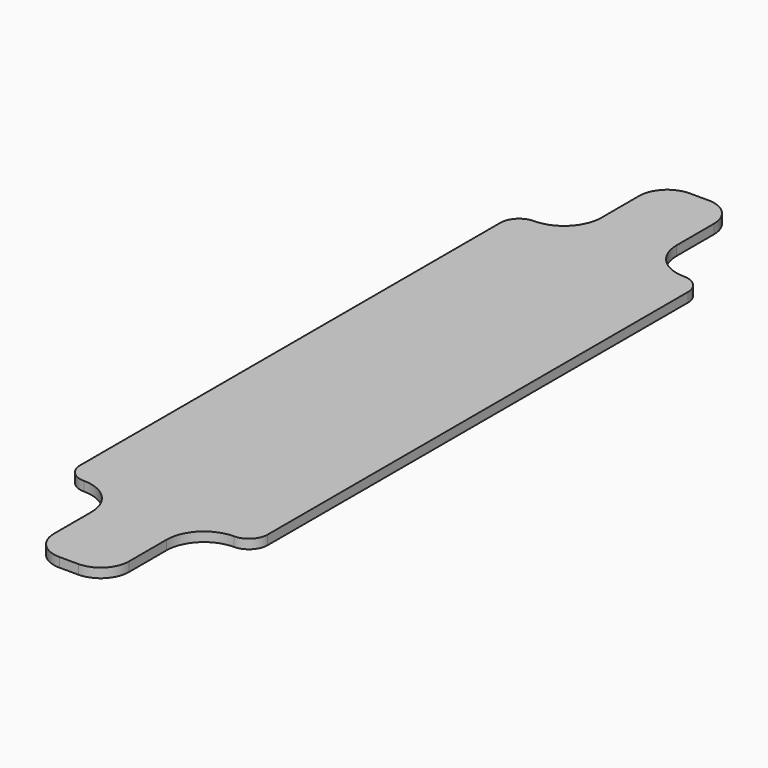
from build123d import *

# Parameters (mm, degrees)
F1_DEPTH = 12.7
F2_R     = 50.8
F3_R     = 38.1
F4_R     = 25.39999


# Not quite as in the source:
# - a fillet or chamfer is up to 0.001 mm smaller than in the source, because OpenCascade refuses the exact size


with BuildPart() as f1:
    # F0 (on Top) → F1 (new body)
    with BuildSketch(Plane.XY):
        Polygon((-50.8, 381), (-127, 381), (-127, 0), (-127, -381), (-50.8, -381), (-50.8, -533.4), (50.8, -533.4), (50.8, -381), (127, -381), (127, 0), (127, 381), (50.8, 381), (50.8, 533.4), (-50.8, 533.4), align=None)
    extrude(amount=F1_DEPTH)

    # F2
    f2_edges = [f1.edges().sort_by_distance(p)[0] for p in [
        (-50.8, 381, 6.35),
        (50.8, 381, 6.35),
        (-50.8, -381, 6.35),
        (50.8, -381, 6.35),
    ]]
    fillet(f2_edges, radius=F2_R)

    # F3
    f3_edges = [f1.edges().sort_by_distance(p)[0] for p in [
        (-50.8, 533.4, 6.35),
        (50.8, 533.4, 6.35),
        (-50.8, -533.4, 6.35),
        (50.8, -533.4, 6.35),
    ]]
    fillet(f3_edges, radius=F3_R)

    # F4 (radius 25.4 in the source; OpenCascade refuses exactly that, so slightly less here)
    f4_edges = [f1.edges().sort_by_distance(p)[0] for p in [
        (-127, 381, 6.35),
        (127, 381, 6.35),
        (127, -381, 6.35),
        (-127, -381, 6.35),
    ]]
    fillet(f4_edges, radius=F4_R)


solid = f1.part
